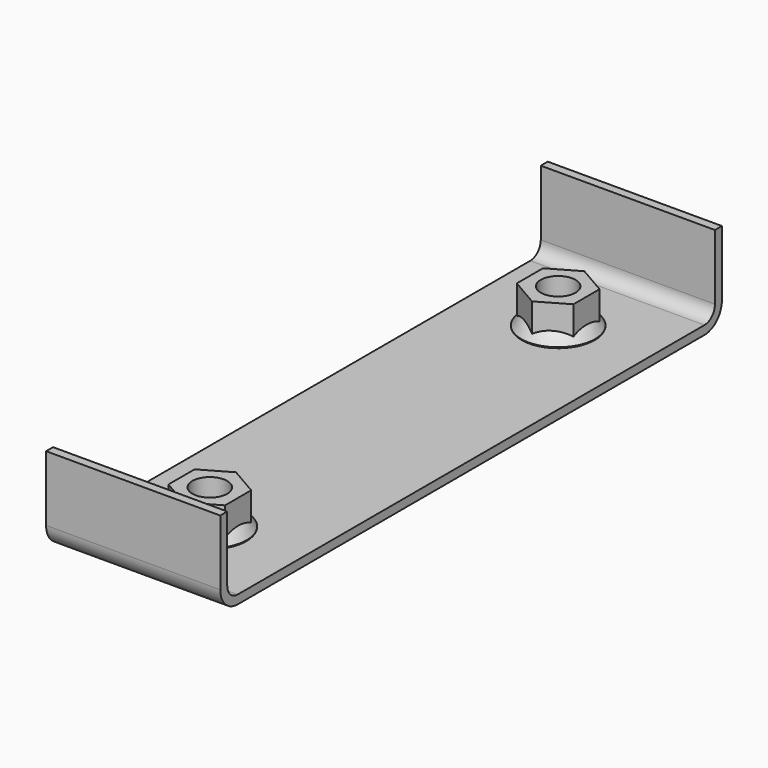
from build123d import *

# Parameters (mm, degrees)
F0_R           = 8.5
F1_DEPTH       = 0.25
F2_DEPTH       = 4
F3_R           = 0.35
F7_DEPTH       = 6
F7_DEPTH_BACK  = 2.25
F8_R           = 4
F9_DEPTH       = 8.251
F11_DEPTH      = 20
F11_DEPTH_BACK = 20
F17_R          = 5
F18_R          = 3
F19_DEPTH      = 25


# Not quite as in the source:
# - a fillet or chamfer that OpenCascade refuses, or shapes differently, is made with other operations: its cross-section is extruded or revolved along the edge and cut away or added


with BuildPart() as f1:
    # F0 (on Top) → F1 (new body)
    with BuildSketch(Plane.XY):
        with Locations((0, 1.1892588809)):
            Circle(F0_R)
    extrude(amount=F1_DEPTH)

    # F2 (add): a face of the model
    f2_faces = [f1.faces().sort_by_distance(p)[0] for p in [
        (0, 1.1892588809, 0.25),
    ]]
    extrude(f2_faces, amount=F2_DEPTH)

    # F3
    f3_edges = [f1.edges().sort_by_distance(p)[0] for p in [
        (-8.5, 1.189259, 0),
    ]]
    fillet(f3_edges, radius=F3_R)

    # F4: fillet of radius 8 on 1 edges, made by hand

    # F4_s1 → F4_t2 (revolve, cut)
    with BuildSketch(Plane.XZ.offset(-1.1892588809)):
        with BuildLine():
            ThreePointArc((8.5, 0.35), (5.5801857334, 3.2070108524), (1.6305022018, 4.25))
            Line((1.6305022018, 4.25), (1.6305022018, 4.41))
            Line((1.6305022018, 4.41), (8.5, 4.41))
            Line((8.5, 4.41), (8.66, 4.25))
            ThreePointArc((8.66, 4.25), (8.66, 2.3), (8.637389956, 0.432))
            Line((8.637389956, 0.432), (8.5, 0.35))
        make_face()
    revolve(axis=Axis((0, 1.1892588809, 4.25), (0, 0, 1)), mode=Mode.SUBTRACT)

    # F6 (on offset) → F7 (join, two sides)
    with BuildSketch(Plane.XY.offset(2.25)) as f7_sk:
        Polygon((-6.5, 4.9420356306), (-6.5, -2.5635178688), (0, -6.3162946186), (6.5, -2.5635178688), (6.5, 4.9420356306), (0, 8.6948123804), align=None)
    extrude(amount=F7_DEPTH)
    extrude(f7_sk.sketch, amount=-F7_DEPTH_BACK)

    # F8 (on face) → F9 (cut, through all)
    with BuildSketch(Plane.XY.offset(8.25)):
        with Locations((0, 1.1892588809)):
            Circle(F8_R)
    extrude(amount=-F9_DEPTH, mode=Mode.SUBTRACT)

    # F10 (on Right) → F11 (join, two sides)
    with BuildSketch(Plane.YZ) as f11_sk:
        Polygon((23.1892588809, 18), (21.1892588809, 18), (21.1892588809, 0), (-118.8107411191, 0), (-118.8107411191, 18), (-120.8107411191, 18), (-120.8107411191, -2), (23.1892588809, -2), align=None)
    extrude(amount=F11_DEPTH)
    extrude(f11_sk.sketch, amount=-F11_DEPTH_BACK)

    # F16: F1 across plane


with BuildPart() as f1_1:
    add(f1.part)
    add(f1.part.mirror(Plane(origin=(-20, -48.8107411191, 0), x_dir=(1, 0, 0), z_dir=(0, -1, 0))))

    # F17
    f17_edges = [f1_1.edges().sort_by_distance(p)[0] for p in [
        (0, 23.189259, -2),
        (0, -120.810741, -2),
    ]]
    fillet(f17_edges, radius=F17_R)

    # F18
    f18_edges = [f1_1.edges().sort_by_distance(p)[0] for p in [
        (0, 21.189259, 0),
        (0, -118.810741, 0),
    ]]
    fillet(f18_edges, radius=F18_R)

    # F19 (cut): faces of the model
    f19_faces = [f1_1.faces().sort_by_distance(p)[0] for p in [
        (0, 1.1892588809, 0),
        (0, -98.8107411191, 0),
    ]]
    extrude(f19_faces, amount=-F19_DEPTH, mode=Mode.SUBTRACT)


solid = f1_1.part
